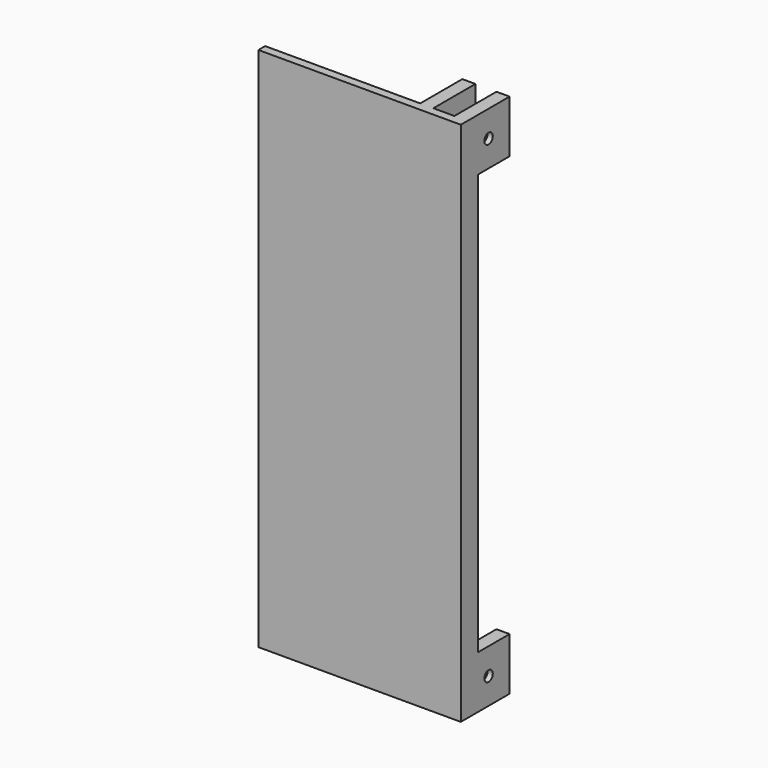
from build123d import *

# Parameters (mm, degrees)
F0_W      = 60
F0_H      = 200
F1_DEPTH  = 3.2
F2_W      = 3
F2_H      = 20
F3_DEPTH  = 20
F5_DEPTH  = 15
F6_DEPTH  = 2
F7_DEPTH  = 2
F8_R      = 2
F9_DEPTH  = 3
F10_DEPTH = 25
F11_R     = 2
F12_DEPTH = 3
F13_DEPTH = 25
F14_W     = 5
F14_H     = 5
F15_DEPTH = 160
F16_W     = 49
F16_H     = 92.5
F17_DEPTH = 1.6


with BuildPart() as f1:
    # F0 (on Front) → F1 (new body)
    with BuildSketch(Plane.XZ):
        with Locations((30, 100)):
            Rectangle(F0_W, F0_H)
    extrude(amount=F1_DEPTH)

    # F2 (on face) → F3 (join)
    with BuildSketch(Plane(origin=(0, 0, 0), x_dir=(-1, 0, 0), z_dir=(0, 1, 0))):
        with Locations((-58.5, 190)):
            Rectangle(F2_W, F2_H)
        with Locations((-58.5, 10)):
            Rectangle(F2_W, F2_H)
        with Locations((-47.5, 190)):
            Rectangle(F2_W, F2_H)
        with Locations((-47.5, 10)):
            Rectangle(F2_W, F2_H)
    extrude(amount=F3_DEPTH)

    # F5 (add): a face of the model
    f5_faces = [f1.faces().sort_by_distance(p)[0] for p in [
        (0, -1.6, 100),
    ]]
    extrude(f5_faces, amount=F5_DEPTH)

    # F6 (add): a face of the model
    f6_faces = [f1.faces().sort_by_distance(p)[0] for p in [
        (60, -1.186588964, 100),
    ]]
    extrude(f6_faces, amount=F6_DEPTH)

    # F7 (add): faces of the model
    f7_faces = [f1.faces().sort_by_distance(p)[0] for p in [
        (46, 10, 190),
        (46, 10, 10),
    ]]
    extrude(f7_faces, amount=F7_DEPTH)

    # F8 (on face) → F9 (cut)
    with BuildSketch(Plane(origin=(57, 0, 0), x_dir=(0, -1, 0), z_dir=(-1, 0, 0))):
        Polygon((-6.7091034656, 10), (-8.3545517328, 12.85), (-11.6454482672, 12.85), (-13.2908965344, 10), (-11.6454482672, 7.15), (-8.3545517328, 7.15), align=None)
        with Locations((-10, 10)):
            Circle(F8_R, mode=Mode.SUBTRACT)
        Polygon((-11.6454482672, 187.15), (-8.3545517328, 187.15), (-6.7091034656, 190), (-8.3545517328, 192.85), (-11.6454482672, 192.85), (-13.2908965344, 190), align=None)
        with Locations((-10, 190)):
            Circle(F8_R, mode=Mode.SUBTRACT)
    extrude(amount=-F9_DEPTH, mode=Mode.SUBTRACT)

    # F10 (cut): faces of the model
    f10_faces = [f1.faces().sort_by_distance(p)[0] for p in [
        (57, 10, 10),
        (57, 10, 190),
    ]]
    extrude(f10_faces, amount=-F10_DEPTH, mode=Mode.SUBTRACT)

    # F11 (on face) → F12 (cut)
    with BuildSketch(Plane(origin=(44, 0, 0), x_dir=(0, -1, 0), z_dir=(-1, 0, 0))):
        Polygon((-6.7091034656, 10), (-8.3545517328, 12.85), (-11.6454482672, 12.85), (-13.2908965344, 10), (-11.6454482672, 7.15), (-8.3545517328, 7.15), align=None)
        with Locations((-10, 10)):
            Circle(F11_R, mode=Mode.SUBTRACT)
        Polygon((-11.6454482672, 187.15), (-8.3545517328, 187.15), (-6.7091034656, 190), (-8.3545517328, 192.85), (-11.6454482672, 192.85), (-13.2908965344, 190), align=None)
        with Locations((-10, 190)):
            Circle(F11_R, mode=Mode.SUBTRACT)
    extrude(amount=-F12_DEPTH, mode=Mode.SUBTRACT)

    # F13 (cut): faces of the model
    f13_faces = [f1.faces().sort_by_distance(p)[0] for p in [
        (44, 10, 190),
        (44, 10, 10),
    ]]
    extrude(f13_faces, amount=-F13_DEPTH, mode=Mode.SUBTRACT)

    # F14 (on face) → F15 (join, through all)
    with BuildSketch(Plane(origin=(0, 0, 180), x_dir=(1, 0, 0), z_dir=(0, 0, -1))):
        with Locations((59.5, -2.5)):
            Rectangle(F14_W, F14_H)
    extrude(amount=F15_DEPTH)

    # F16 (on face) → F17 (cut)
    with BuildSketch(Plane(origin=(0, 0, 0), x_dir=(-1, 0, 0), z_dir=(0, 1, 0))):
        with Locations((-14.5, 51.25)):
            Rectangle(F16_W, F16_H)
        with Locations((-14.5, 148.75)):
            Rectangle(F16_W, F16_H)
    extrude(amount=-F17_DEPTH, mode=Mode.SUBTRACT)


solid = f1.part
